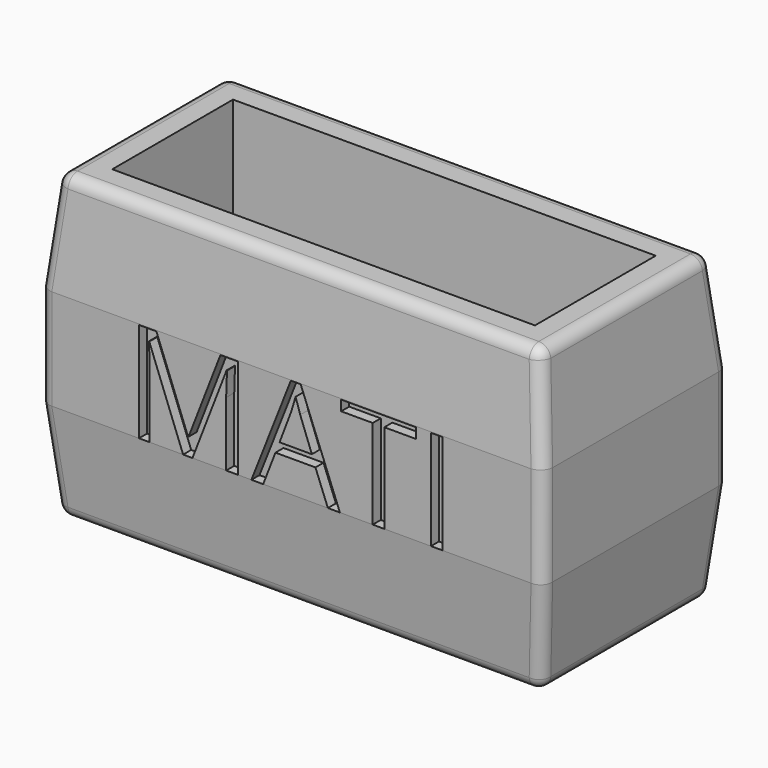
from build123d import *

# Parameters (mm, degrees)
F0_W          = 24.9999998945
F0_H          = 11.4999998945
F0_W_2        = 21
F0_H_2        = 7.5
F1_DEPTH      = 15
F2_SIZE2      = 0.5
F2_SIZE       = 5
F3_SIZE2      = 5
F3_SIZE       = 0.5
F4_T1_DEPTH   = 22.91401482
F4_T3_DEPTH   = 9.41401482
F4_T5_DEPTH   = 11.989299061
F4_T7_DEPTH   = 20
F4_T9_DEPTH   = 11.989299061
F4_T11_DEPTH  = 11.989299061
F4_T13_DEPTH  = 11.989299061
F4_T15_DEPTH  = 11.989299061
F4_T17_DEPTH  = 11.989299061
F4_T19_DEPTH  = 11.989299061
F4_T21_DEPTH  = 11.989299061
F4_T26_DEPTH  = 1.1694194197
F4_S37_W      = 2.3388388394
F4_S37_H      = 2.3388388393
F4_T38_DEPTH  = 1.1694194197
F4_S49_W      = 2.3388388393
F4_S49_H      = 2.3388388393
F4_T50_DEPTH  = 1.1694194197
F4_S61_W      = 2.3388388394
F4_S61_H      = 2.3388388394
F4_T62_DEPTH  = 1.1694194197
F4_S73_W      = 2.3388388394
F4_S73_H      = 2.3388388393
F4_T74_DEPTH  = 1.1694194197
F4_S85_W      = 2.3388388393
F4_S85_H      = 2.3388388393
F4_T86_DEPTH  = 1.1694194197
F4_S97_W      = 2.3388388394
F4_S97_H      = 2.3388388394
F4_T98_DEPTH  = 1.1694194197
F4_S109_W     = 2.3388388394
F4_S109_H     = 2.3388388394
F4_T110_DEPTH = 1.1694194197
F5_TEXT_SIZE  = 6.9444444444
F6_DEPTH      = 0.5


# Not quite as in the source:
# - a fillet or chamfer that OpenCascade refuses, or shapes differently, is made with other operations: its cross-section is extruded or revolved along the edge and cut away or added
# - Text() gives the source's letters only with a copy of the font that has no kerning and outlines rounded to 1/6400 em; it was checked with that copy


with BuildPart() as f1:
    # F0 (on Top) → F1 (new body)
    with BuildSketch(Plane.XY):
        with Locations((0.4532363685, -0.9334524454)):
            Rectangle(F0_W, F0_H)
        with Locations((0.4532363685, -0.9334524454)):
            Rectangle(F0_W_2, F0_H_2, mode=Mode.SUBTRACT)
    extrude(amount=F1_DEPTH)

    # F2
    f2_edges = [f1.edges().sort_by_distance(p)[0] for p in [
        (0.453236, 4.816548, 15),
        (12.953236, -0.933452, 15),
        (0.453236, -6.683452, 15),
        (-12.046764, -0.933452, 15),
    ]]
    chamfer(f2_edges, length=F2_SIZE, length2=F2_SIZE2)

    # F3
    f3_edges = [f1.edges().sort_by_distance(p)[0] for p in [
        (12.953236, -0.933452, 0),
        (0.453236, 4.816548, 0),
        (-12.046764, -0.933452, 0),
        (0.453236, -6.683452, 0),
    ]]
    f3_side = f1.faces().sort_by_distance((12.678055, -0.933452, 0))[0]
    chamfer(f3_edges, length=F3_SIZE, length2=F3_SIZE2, reference=f3_side)

    # F4: fillet of radius 0.6 on 20 edges, made by hand

    # F4_s2 → F4_t1 (cut)
    with BuildSketch(Plane.YZ.offset(-11.0037710415)):
        with BuildLine():
            ThreePointArc((3.7735549646, 15), (4.176158157, 14.8448715201), (4.3705772787, 14.4597022314))
            Line((4.3705772787, 14.4597022314), (4.3165475018, 15))
            Line((4.3165475018, 15), (3.7735549646, 15))
        make_face()
        with BuildLine():
            ThreePointArc((-6.2374821696, 14.4597022314), (-6.0430630479, 14.8448715201), (-5.6404598554, 15))
            Line((-5.6404598554, 15), (-6.1834523927, 15))
            Line((-6.1834523927, 15), (-6.2374821696, 14.4597022314))
        make_face()
        with BuildLine():
            ThreePointArc((3.7735549646, 0), (4.176158157, 0.1551284799), (4.3705772787, 0.5402977686))
            Line((4.3705772787, 0.5402977686), (4.3165475018, 0))
            Line((4.3165475018, 0), (3.7735549646, 0))
        make_face()
        with BuildLine():
            ThreePointArc((-6.2374821696, 0.5402977686), (-6.0430630479, 0.1551284799), (-5.6404598554, 0))
            Line((-5.6404598554, 0), (-6.1834523927, 0))
            Line((-6.1834523927, 0), (-6.2374821696, 0.5402977686))
        make_face()
    extrude(amount=F4_T1_DEPTH, mode=Mode.SUBTRACT)

    # F4_s4 → F4_t3 (cut)
    with BuildSketch(Plane.XZ.offset(-3.7735549646)):
        with BuildLine():
            ThreePointArc((12.5072660926, 14.4597022314), (12.3128469709, 14.8448715201), (11.9102437785, 15))
            Line((11.9102437785, 15), (12.4532363157, 15))
            Line((12.4532363157, 15), (12.5072660926, 14.4597022314))
        make_face()
        with BuildLine():
            ThreePointArc((-11.0037710415, 15), (-11.406374234, 14.8448715201), (-11.6007933557, 14.4597022314))
            Line((-11.6007933557, 14.4597022314), (-11.5467635788, 15))
            Line((-11.5467635788, 15), (-11.0037710415, 15))
        make_face()
        with BuildLine():
            ThreePointArc((12.5072660926, 0.5402977686), (12.3128469709, 0.1551284799), (11.9102437785, 0))
            Line((11.9102437785, 0), (12.4532363157, 0))
            Line((12.4532363157, 0), (12.5072660926, 0.5402977686))
        make_face()
        with BuildLine():
            ThreePointArc((-11.0037710415, 0), (-11.406374234, 0.1551284799), (-11.6007933557, 0.5402977686))
            Line((-11.6007933557, 0.5402977686), (-11.5467635788, 0))
            Line((-11.5467635788, 0), (-11.0037710415, 0))
        make_face()
    extrude(amount=F4_T3_DEPTH, mode=Mode.SUBTRACT)

    # F4_s6 → F4_t5 (cut)
    with BuildSketch(Plane(origin=(0.0614684709, 0.0614684709, 0.6146847087), x_dir=(-0.7071067812, 0.7071067812, 0), z_dir=(0.0990147543, 0.0990147543, 0.990147543))):
        with BuildLine():
            ThreePointArc((3.3702751825, 14.0960550532), (3.7924337093, 14.2696958405), (4.2145922362, 14.0960550532))
            Line((4.2145922362, 14.0960550532), (3.7924337093, 14.5140542813))
            Line((3.7924337093, 14.5140542813), (3.3702751825, 14.0960550532))
        make_face()
    extrude(amount=F4_T5_DEPTH, mode=Mode.SUBTRACT)

    # F4_s8 → F4_t7 (cut)
    with BuildSketch(Plane.XY.offset(-2.5)):
        with BuildLine():
            ThreePointArc((-11.4467635788, -6.6834523927), (-11.8710276475, -6.5077164614), (-12.0467635788, -6.0834523927))
            Line((-12.0467635788, -6.0834523927), (-12.0467635788, -6.6834523927))
            Line((-12.0467635788, -6.6834523927), (-11.4467635788, -6.6834523927))
        make_face()
        with BuildLine():
            ThreePointArc((12.9532363157, -6.0834523927), (12.7775003844, -6.5077164614), (12.3532363157, -6.6834523927))
            Line((12.3532363157, -6.6834523927), (12.9532363157, -6.6834523927))
            Line((12.9532363157, -6.6834523927), (12.9532363157, -6.0834523927))
        make_face()
        with BuildLine():
            ThreePointArc((12.9532363157, 4.2165475018), (12.7775003844, 4.6408115705), (12.3532363157, 4.8165475018))
            Line((12.3532363157, 4.8165475018), (12.9532363157, 4.8165475018))
            Line((12.9532363157, 4.8165475018), (12.9532363157, 4.2165475018))
        make_face()
        with BuildLine():
            ThreePointArc((-11.4467635788, 4.8165475018), (-11.8710276475, 4.6408115705), (-12.0467635788, 4.2165475018))
            Line((-12.0467635788, 4.2165475018), (-12.0467635788, 4.8165475018))
            Line((-12.0467635788, 4.8165475018), (-11.4467635788, 4.8165475018))
        make_face()
    extrude(amount=F4_T7_DEPTH, mode=Mode.SUBTRACT)

    # F4_s10 → F4_t9 (cut)
    with BuildSketch(Plane(origin=(-0.2220022637, -0.2220022637, 2.220022637), x_dir=(0.7071067812, -0.7071067812, 0), z_dir=(-0.0990147543, -0.0990147543, 0.990147543))):
        with BuildLine():
            ThreePointArc((-3.3702751825, -11.9956349271), (-3.7924337093, -12.1692757145), (-4.2145922362, -11.9956349271))
            Line((-4.2145922362, -11.9956349271), (-3.7924337093, -12.4136341552))
            Line((-3.7924337093, -12.4136341552), (-3.3702751825, -11.9956349271))
        make_face()
    extrude(amount=F4_T9_DEPTH, mode=Mode.SUBTRACT)

    # F4_s12 → F4_t11 (cut)
    with BuildSketch(Plane(origin=(-0.0525814833, 0.0525814833, 0.5258148325), x_dir=(-0.7071067812, -0.7071067812, 0), z_dir=(-0.0990147543, 0.0990147543, 0.990147543))):
        with BuildLine():
            ThreePointArc((-4.8555652554, 14.7307129133), (-4.4334067285, 14.9043537006), (-4.0112482017, 14.7307129133))
            Line((-4.0112482017, 14.7307129133), (-4.4334067285, 15.1487121414))
            Line((-4.4334067285, 15.1487121414), (-4.8555652554, 14.7307129133))
        make_face()
    extrude(amount=F4_T11_DEPTH, mode=Mode.SUBTRACT)

    # F4_s14 → F4_t13 (cut)
    with BuildSketch(Plane(origin=(0.2308892513, -0.2308892513, 2.3088925131), x_dir=(0.7071067812, 0.7071067812, 0), z_dir=(0.0990147543, -0.0990147543, 0.990147543))):
        with BuildLine():
            ThreePointArc((4.8555652554, -12.6302927872), (4.4334067285, -12.8039335746), (4.0112482017, -12.6302927872))
            Line((4.0112482017, -12.6302927872), (4.4334067285, -13.0482920153))
            Line((4.4334067285, -13.0482920153), (4.8555652554, -12.6302927872))
        make_face()
    extrude(amount=F4_T13_DEPTH, mode=Mode.SUBTRACT)

    # F4_s16 → F4_t15 (cut)
    with BuildSketch(Plane(origin=(-0.0708844724, -0.0708844724, 0.7088447238), x_dir=(0.7071067812, -0.7071067812, 0), z_dir=(-0.0990147543, -0.0990147543, 0.990147543))):
        with BuildLine():
            ThreePointArc((6.1756663635, 13.4236180445), (5.7535078367, 13.5972588319), (5.3313493099, 13.4236180445))
            Line((5.3313493099, 13.4236180445), (5.7535078367, 13.8416172726))
            Line((5.7535078367, 13.8416172726), (6.1756663635, 13.4236180445))
        make_face()
    extrude(amount=F4_T15_DEPTH, mode=Mode.SUBTRACT)

    # F4_s18 → F4_t17 (cut)
    with BuildSketch(Plane(origin=(0.2125862622, 0.2125862622, 2.1258626219), x_dir=(-0.7071067812, 0.7071067812, 0), z_dir=(0.0990147543, 0.0990147543, 0.990147543))):
        with BuildLine():
            ThreePointArc((-6.1756663635, -11.3231979185), (-5.7535078367, -11.4968387058), (-5.3313493099, -11.3231979185))
            Line((-5.3313493099, -11.3231979185), (-5.7535078367, -11.7411971466))
            Line((-5.7535078367, -11.7411971466), (-6.1756663635, -11.3231979185))
        make_face()
    extrude(amount=F4_T17_DEPTH, mode=Mode.SUBTRACT)

    # F4_s20 → F4_t19 (cut)
    with BuildSketch(Plane(origin=(0.07977146, -0.07977146, 0.7977145999), x_dir=(0.7071067812, 0.7071067812, 0), z_dir=(0.0990147543, -0.0990147543, 0.990147543))):
        with BuildLine():
            ThreePointArc((-4.6903762906, 12.7889601844), (-5.1125348175, 12.9626009718), (-5.5346933443, 12.7889601844))
            Line((-5.5346933443, 12.7889601844), (-5.1125348175, 13.2069594125))
            Line((-5.1125348175, 13.2069594125), (-4.6903762906, 12.7889601844))
        make_face()
    extrude(amount=F4_T19_DEPTH, mode=Mode.SUBTRACT)

    # F4_s22 → F4_t21 (cut)
    with BuildSketch(Plane(origin=(-0.2036992746, 0.2036992746, 2.0369927457), x_dir=(-0.7071067812, -0.7071067812, 0), z_dir=(-0.0990147543, 0.0990147543, 0.990147543))):
        with BuildLine():
            ThreePointArc((4.6903762906, -10.6885400584), (5.1125348175, -10.8621808457), (5.5346933443, -10.6885400584))
            Line((5.5346933443, -10.6885400584), (5.1125348175, -11.1065392865))
            Line((5.1125348175, -11.1065392865), (4.6903762906, -10.6885400584))
        make_face()
    extrude(amount=F4_T21_DEPTH, mode=Mode.SUBTRACT)


with BuildPart() as f4_tool24:
    # F4_s25 → F4_t26 (new body)
    with BuildSketch(Plane(origin=(9.5700078939, 9.5700078939, 11.5317404815), x_dir=(-0.7071067812, 0.7071067812, 0), z_dir=(0.538226305, 0.538226305, 0.6485560031))):
        Polygon((-7.3384679014, 4.2404527838), (-6.2257208728, 2.1832796829), (-4.168547772, 3.2960267116), (-5.2812948006, 5.3531998124), align=None)
    extrude(amount=F4_T26_DEPTH)

    split(bisect_by=Plane.XZ.offset(-3.7735549646), keep=Keep.BOTTOM)

    split(bisect_by=Plane.YZ.offset(11.9102437785), keep=Keep.TOP)

    split(bisect_by=Plane(origin=(-1.2580019731, -1.2580019731, 12.5800197311), x_dir=(0.7071067812, -0.7071067812, 0), z_dir=(-0.0990147543, -0.0990147543, 0.990147543)), keep=Keep.TOP)

    split(bisect_by=Plane(origin=(13.8150854611, 0, 1.3815085461), x_dir=(0, 1, 0), z_dir=(-0.9950371902, 0, -0.099503719)), keep=Keep.TOP)

    split(bisect_by=Plane.XY.offset(15), keep=Keep.BOTTOM)

    split(bisect_by=Plane(origin=(0, 5.7589579226, 0.5758957923), x_dir=(1, 0, 0), z_dir=(0, -0.9950371902, -0.099503719)), keep=Keep.TOP)

    # F4_s33 → F4_t34 (revolve, cut)
    with BuildSketch(Plane(origin=(11.9102437785, 3.7735549646, 14.4), x_dir=(-0.538226305, -0.538226305, -0.6485560031), z_dir=(0.8401369797, -0.40376322, -0.3621396382))):
        with BuildLine():
            ThreePointArc((0, -0.6), (0.6, 0), (0, 0.6))
            Line((0, 0.6), (0, -0.6))
        make_face()
    revolve(axis=Axis((11.9102437785, 3.7735549646, 14.4), (0.0669499808, 0.739788961, -0.6694998083)), mode=Mode.SUBTRACT)


with BuildPart() as f1_1:
    add(f1.part)

    # F4_t23: cut F4_tool24
    add(f4_tool24.part, mode=Mode.SUBTRACT)


with BuildPart() as f4_tool36:
    # F4_s37 → F4_t38 (new body)
    with BuildSketch(Plane(origin=(-9.3074140227, 9.3074140227, 11.2153181328), x_dir=(-0.7071067812, -0.7071067812, 0), z_dir=(-0.538226305, 0.538226305, 0.6485560031))):
        with Locations((5.1125348175, 4.1839466471)):
            Rectangle(F4_S37_W, F4_S37_H)
    extrude(amount=F4_T38_DEPTH)

    split(bisect_by=Plane.YZ.offset(-11.0037710415), keep=Keep.BOTTOM)

    split(bisect_by=Plane(origin=(1.2668889607, -1.2668889607, 12.6688896072), x_dir=(0.7071067812, 0.7071067812, 0), z_dir=(0.0990147543, -0.0990147543, 0.990147543)), keep=Keep.TOP)

    split(bisect_by=Plane.XZ.offset(-3.7735549646), keep=Keep.BOTTOM)

    split(bisect_by=Plane.XY.offset(15), keep=Keep.BOTTOM)

    split(bisect_by=Plane(origin=(0, 5.7589579226, 0.5758957923), x_dir=(1, 0, 0), z_dir=(0, -0.9950371902, -0.099503719)), keep=Keep.TOP)

    split(bisect_by=Plane(origin=(-12.9175877018, 0, 1.2917587702), x_dir=(0, 1, 0), z_dir=(0.9950371902, 0, -0.099503719)), keep=Keep.TOP)

    # F4_s45 → F4_t46 (revolve, cut)
    with BuildSketch(Plane(origin=(-11.0037710415, 3.7735549646, 14.4), x_dir=(0.538226305, -0.538226305, -0.6485560031), z_dir=(0.4585983478, -0.4585983478, 0.7611669402))):
        with BuildLine():
            ThreePointArc((0, -0.6), (0.6, 0), (0, 0.6))
            Line((0, 0.6), (0, -0.6))
        make_face()
    revolve(axis=Axis((-11.0037710415, 3.7735549646, 14.4), (0.7071067812, 0.7071067812, 0)), mode=Mode.SUBTRACT)


with BuildPart() as f1_2:
    add(f1_1.part)

    # F4_t35: cut F4_tool36
    add(f4_tool36.part, mode=Mode.SUBTRACT)


with BuildPart() as f4_tool48:
    # F4_s49 → F4_t50 (new body)
    with BuildSketch(Plane(origin=(10.1108270079, -10.1108270079, 12.1834207872), x_dir=(0.7071067812, 0.7071067812, 0), z_dir=(0.538226305, -0.538226305, 0.6485560031))):
        with Locations((4.4334067286, 2.9120802493)):
            Rectangle(F4_S49_W, F4_S49_H)
    extrude(amount=F4_T50_DEPTH)

    split(bisect_by=Plane.XZ.offset(5.6404598554), keep=Keep.TOP)

    split(bisect_by=Plane(origin=(-1.239698984, 1.239698984, 12.3969898398), x_dir=(-0.7071067812, -0.7071067812, 0), z_dir=(-0.0990147543, 0.0990147543, 0.990147543)), keep=Keep.TOP)

    split(bisect_by=Plane.YZ.offset(11.9102437785), keep=Keep.TOP)

    split(bisect_by=Plane.XY.offset(15), keep=Keep.BOTTOM)

    split(bisect_by=Plane(origin=(13.8150854611, 0, 1.3815085461), x_dir=(0, 1, 0), z_dir=(-0.9950371902, 0, -0.099503719)), keep=Keep.TOP)

    split(bisect_by=Plane(origin=(0, -7.6073786066, 0.7607378607), x_dir=(1, 0, 0), z_dir=(0, 0.9950371902, -0.099503719)), keep=Keep.TOP)

    # F4_s57 → F4_t58 (revolve, cut)
    with BuildSketch(Plane(origin=(11.9102437785, -5.6404598554, 14.4), x_dir=(-0.538226305, 0.538226305, -0.6485560031), z_dir=(-0.4585983478, 0.4585983478, 0.7611669402))):
        with BuildLine():
            ThreePointArc((0, -0.6), (0.6, 0), (0, 0.6))
            Line((0, 0.6), (0, -0.6))
        make_face()
    revolve(axis=Axis((11.9102437785, -5.6404598554, 14.4), (-0.7071067812, -0.7071067812, 0)), mode=Mode.SUBTRACT)


with BuildPart() as f1_3:
    add(f1_2.part)

    # F4_t47: cut F4_tool48
    add(f4_tool48.part, mode=Mode.SUBTRACT)


with BuildPart() as f4_tool60:
    # F4_s61 → F4_t62 (new body)
    with BuildSketch(Plane(origin=(-9.8482331367, -9.8482331367, 11.8669984385), x_dir=(0.7071067812, -0.7071067812, 0), z_dir=(-0.538226305, -0.538226305, 0.6485560031))):
        with Locations((-3.7924337093, 3.3277871487)):
            Rectangle(F4_S61_W, F4_S61_H)
    extrude(amount=F4_T62_DEPTH)

    split(bisect_by=Plane.XZ.offset(5.6404598554), keep=Keep.TOP)

    split(bisect_by=Plane(origin=(1.2485859716, 1.2485859716, 12.485859716), x_dir=(-0.7071067812, 0.7071067812, 0), z_dir=(0.0990147543, 0.0990147543, 0.990147543)), keep=Keep.TOP)

    split(bisect_by=Plane.YZ.offset(-11.0037710415), keep=Keep.BOTTOM)

    split(bisect_by=Plane.XY.offset(15), keep=Keep.BOTTOM)

    split(bisect_by=Plane(origin=(-12.9175877018, 0, 1.2917587702), x_dir=(0, 1, 0), z_dir=(0.9950371902, 0, -0.099503719)), keep=Keep.TOP)

    split(bisect_by=Plane(origin=(0, -7.6073786066, 0.7607378607), x_dir=(1, 0, 0), z_dir=(0, 0.9950371902, -0.099503719)), keep=Keep.TOP)

    # F4_s69 → F4_t70 (revolve, cut)
    with BuildSketch(Plane(origin=(-11.0037710415, -5.6404598554, 14.4), x_dir=(0.538226305, 0.538226305, -0.6485560031), z_dir=(0.4585983478, 0.4585983478, 0.7611669402))):
        with BuildLine():
            ThreePointArc((0, -0.6), (0.6, 0), (0, 0.6))
            Line((0, 0.6), (0, -0.6))
        make_face()
    revolve(axis=Axis((-11.0037710415, -5.6404598554, 14.4), (-0.7071067812, 0.7071067812, 0)), mode=Mode.SUBTRACT)


with BuildPart() as f1_4:
    add(f1_3.part)

    # F4_t59: cut F4_tool60
    add(f4_tool60.part, mode=Mode.SUBTRACT)


with BuildPart() as f4_tool72:
    # F4_s73 → F4_t74 (new body)
    with BuildSketch(Plane(origin=(-4.6121846194, -4.6121846194, -5.5576251005), x_dir=(0.7071067812, -0.7071067812, 0), z_dir=(-0.538226305, -0.538226305, -0.6485560031))):
        with Locations((-3.7924337093, 8.0897169538)):
            Rectangle(F4_S73_W, F4_S73_H)
    extrude(amount=F4_T74_DEPTH)

    split(bisect_by=Plane.XZ.offset(5.6404598554), keep=Keep.TOP)

    split(bisect_by=Plane(origin=(-0.2220022637, -0.2220022637, 2.220022637), x_dir=(-0.7071067812, 0.7071067812, 0), z_dir=(0.0990147543, 0.0990147543, -0.990147543)), keep=Keep.TOP)

    split(bisect_by=Plane.YZ.offset(-11.0037710415), keep=Keep.BOTTOM)

    split(bisect_by=Plane.XY, keep=Keep.TOP)

    split(bisect_by=Plane(origin=(-11.4324391869, 0, -1.1432439187), x_dir=(0, 1, 0), z_dir=(0.9950371902, 0, 0.099503719)), keep=Keep.TOP)

    split(bisect_by=Plane(origin=(0, -6.1222300918, -0.6122230092), x_dir=(1, 0, 0), z_dir=(0, 0.9950371902, 0.099503719)), keep=Keep.TOP)

    # F4_s81 → F4_t82 (revolve, cut)
    with BuildSketch(Plane(origin=(-11.0037710415, -5.6404598554, 0.6), x_dir=(0.538226305, 0.538226305, 0.6485560031), z_dir=(0.4585983478, 0.4585983478, -0.7611669402))):
        with BuildLine():
            ThreePointArc((0, -0.6), (0.6, 0), (0, 0.6))
            Line((0, 0.6), (0, -0.6))
        make_face()
    revolve(axis=Axis((-11.0037710415, -5.6404598554, 0.6), (0.7071067812, -0.7071067812, 0)), mode=Mode.SUBTRACT)


with BuildPart() as f1_5:
    add(f1_4.part)

    # F4_t71: cut F4_tool72
    add(f4_tool72.part, mode=Mode.SUBTRACT)


with BuildPart() as f4_tool84:
    # F4_s85 → F4_t86 (new body)
    with BuildSketch(Plane(origin=(4.8747784906, -4.8747784906, -5.8740474492), x_dir=(0.7071067812, 0.7071067812, 0), z_dir=(0.538226305, -0.538226305, -0.6485560031))):
        with Locations((4.4334067286, 8.5054238533)):
            Rectangle(F4_S85_W, F4_S85_H)
    extrude(amount=F4_T86_DEPTH)

    split(bisect_by=Plane.XZ.offset(5.6404598554), keep=Keep.TOP)

    split(bisect_by=Plane(origin=(0.2308892513, -0.2308892513, 2.3088925131), x_dir=(-0.7071067812, -0.7071067812, 0), z_dir=(-0.0990147543, 0.0990147543, -0.990147543)), keep=Keep.TOP)

    split(bisect_by=Plane.YZ.offset(11.9102437785), keep=Keep.TOP)

    split(bisect_by=Plane.XY, keep=Keep.TOP)

    split(bisect_by=Plane(origin=(12.3299369463, 0, -1.2329936946), x_dir=(0, 1, 0), z_dir=(-0.9950371902, 0, 0.099503719)), keep=Keep.TOP)

    split(bisect_by=Plane(origin=(0, -6.1222300918, -0.6122230092), x_dir=(1, 0, 0), z_dir=(0, 0.9950371902, 0.099503719)), keep=Keep.TOP)

    # F4_s93 → F4_t94 (revolve, cut)
    with BuildSketch(Plane(origin=(11.9102437785, -5.6404598554, 0.6), x_dir=(-0.538226305, 0.538226305, 0.6485560031), z_dir=(-0.4585983478, 0.4585983478, -0.7611669402))):
        with BuildLine():
            ThreePointArc((0, -0.6), (0.6, 0), (0, 0.6))
            Line((0, 0.6), (0, -0.6))
        make_face()
    revolve(axis=Axis((11.9102437785, -5.6404598554, 0.6), (0.7071067812, 0.7071067812, 0)), mode=Mode.SUBTRACT)


with BuildPart() as f1_6:
    add(f1_5.part)

    # F4_t83: cut F4_tool84
    add(f4_tool84.part, mode=Mode.SUBTRACT)


with BuildPart() as f4_tool96:
    # F4_s97 → F4_t98 (new body)
    with BuildSketch(Plane(origin=(4.3339593766, 4.3339593766, -5.2223671434), x_dir=(-0.7071067812, 0.7071067812, 0), z_dir=(0.538226305, 0.538226305, -0.6485560031))):
        with Locations((-5.7535078367, 7.6492643548)):
            Rectangle(F4_S97_W, F4_S97_H)
    extrude(amount=F4_T98_DEPTH)

    split(bisect_by=Plane.YZ.offset(11.9102437785), keep=Keep.TOP)

    split(bisect_by=Plane(origin=(0.2125862622, 0.2125862622, 2.1258626219), x_dir=(0.7071067812, -0.7071067812, 0), z_dir=(-0.0990147543, -0.0990147543, -0.990147543)), keep=Keep.TOP)

    split(bisect_by=Plane.XZ.offset(-3.7735549646), keep=Keep.BOTTOM)

    split(bisect_by=Plane.XY, keep=Keep.TOP)

    split(bisect_by=Plane(origin=(0, 4.2738094078, -0.4273809408), x_dir=(1, 0, 0), z_dir=(0, -0.9950371902, 0.099503719)), keep=Keep.TOP)

    split(bisect_by=Plane(origin=(12.3299369463, 0, -1.2329936946), x_dir=(0, 1, 0), z_dir=(-0.9950371902, 0, 0.099503719)), keep=Keep.TOP)

    # F4_s105 → F4_t106 (revolve, cut)
    with BuildSketch(Plane(origin=(11.9102437785, 3.7735549646, 0.6), x_dir=(-0.538226305, -0.538226305, 0.6485560031), z_dir=(-0.4585983478, -0.4585983478, -0.7611669402))):
        with BuildLine():
            ThreePointArc((0, -0.6), (0.6, 0), (0, 0.6))
            Line((0, 0.6), (0, -0.6))
        make_face()
    revolve(axis=Axis((11.9102437785, 3.7735549646, 0.6), (-0.7071067812, 0.7071067812, 0)), mode=Mode.SUBTRACT)


with BuildPart() as f1_7:
    add(f1_6.part)

    # F4_t95: cut F4_tool96
    add(f4_tool96.part, mode=Mode.SUBTRACT)


with BuildPart() as f4_tool108:
    # F4_s109 → F4_t110 (new body)
    with BuildSketch(Plane(origin=(-4.0713655054, 4.0713655054, -4.9059447948), x_dir=(-0.7071067812, -0.7071067812, 0), z_dir=(-0.538226305, 0.538226305, -0.6485560031))):
        with Locations((5.1125348175, 7.2335574553)):
            Rectangle(F4_S109_W, F4_S109_H)
    extrude(amount=F4_T110_DEPTH)

    split(bisect_by=Plane.YZ.offset(-11.0037710415), keep=Keep.BOTTOM)

    split(bisect_by=Plane(origin=(-0.2036992746, 0.2036992746, 2.0369927457), x_dir=(0.7071067812, 0.7071067812, 0), z_dir=(0.0990147543, -0.0990147543, -0.990147543)), keep=Keep.TOP)

    split(bisect_by=Plane.XZ.offset(-3.7735549646), keep=Keep.BOTTOM)

    split(bisect_by=Plane.XY, keep=Keep.TOP)

    split(bisect_by=Plane(origin=(0, 4.2738094078, -0.4273809408), x_dir=(1, 0, 0), z_dir=(0, -0.9950371902, 0.099503719)), keep=Keep.TOP)

    split(bisect_by=Plane(origin=(-11.4324391869, 0, -1.1432439187), x_dir=(0, 1, 0), z_dir=(0.9950371902, 0, 0.099503719)), keep=Keep.TOP)

    # F4_s117 → F4_t118 (revolve, cut)
    with BuildSketch(Plane(origin=(-11.0037710415, 3.7735549646, 0.6), x_dir=(0.538226305, -0.538226305, 0.6485560031), z_dir=(0.4585983478, -0.4585983478, -0.7611669402))):
        with BuildLine():
            ThreePointArc((0, -0.6), (0.6, 0), (0, 0.6))
            Line((0, 0.6), (0, -0.6))
        make_face()
    revolve(axis=Axis((-11.0037710415, 3.7735549646, 0.6), (-0.7071067812, -0.7071067812, 0)), mode=Mode.SUBTRACT)


with BuildPart() as f1_8:
    add(f1_7.part)

    # F4_t107: cut F4_tool108
    add(f4_tool108.part, mode=Mode.SUBTRACT)

    # F5 (on face) → F6 (cut)
    with BuildSketch(Plane.XZ.offset(6.6834523927)):
        with Locations((-7.8023239039, 5)):
            Text('MATI', F5_TEXT_SIZE, font='Open Sans', text_align=(TextAlign.LEFT, TextAlign.BOTTOM))
    extrude(amount=-F6_DEPTH, mode=Mode.SUBTRACT)


solid = f1_8.part
